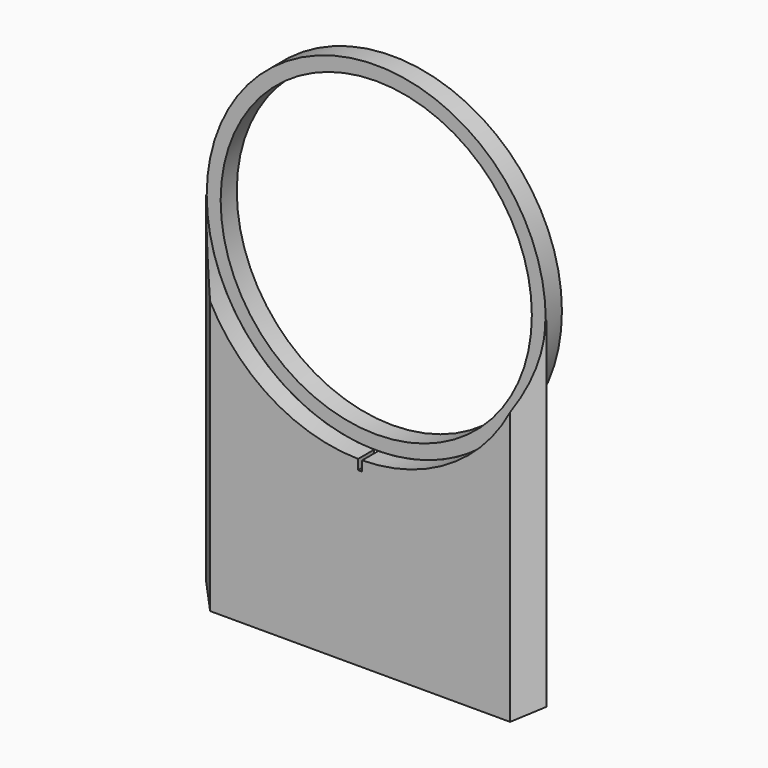
from build123d import *

# Parameters (mm, degrees)
F1_R         = 42.0358065459
F3_DEPTH     = 5
F2_R         = 38.5790977184
F4_DEPTH     = 5
F0_R         = 2
F5_DEPTH     = 25
F6_W         = 84.3785708158
F6_H         = 87.1892854079
F6_W_2       = 1
F6_H_2       = 5
F7_DEPTH     = 5
F8_DEPTH     = 5
F9_SIZE2     = 2.886741
F9_SIZE      = 4.99999
F10_T1_DEPTH = 112.9061152876


# Not quite as in the source:
# - a fillet or chamfer that OpenCascade refuses, or shapes differently, is made with other operations: its cross-section is extruded or revolved along the edge and cut away or added
# - a fillet or chamfer is up to 0.001 mm smaller than in the source, because OpenCascade refuses the exact size


with BuildPart() as f3:
    # F1 (on Front) → F3 (new body, symmetric)
    with BuildSketch(Plane.XZ):
        Circle(F1_R)
    extrude(amount=F3_DEPTH, both=True)

    # F2 (on Front) → F4 (cut)
    with BuildSketch(Plane.XZ):
        Circle(F2_R)
    extrude(amount=-F4_DEPTH, mode=Mode.SUBTRACT)

    # F0 (on Front) → F5 (cut)
    with BuildSketch(Plane.XZ):
        with BuildLine():
            ThreePointArc((26, 24), (24, 26), (22, 24))
            ThreePointArc((22, 24), (24, 22), (26, 24))
        make_face()
        with BuildLine():
            ThreePointArc((12.5, 24), (0, 27.0601182555), (-12.5, 24))
            Line((-12.5, 24), (12.5, 24))
        make_face()
        with BuildLine():
            Line((12.5, 24), (-12.5, 24))
            ThreePointArc((-12.5, 24), (-27.0601182555, 0), (-12.5, -24))
            Line((-12.5, -24), (12.5, -24))
            ThreePointArc((12.5, -24), (23.1354865757, -14.0356425184), (27.0601182555, 0))
            ThreePointArc((27.0601182555, 0), (23.1354865757, 14.0356425184), (12.5, 24))
        make_face()
        with Locations((-24, 24)):
            Circle(F0_R)
        with BuildLine():
            ThreePointArc((12.5, -24), (0, -27.0601182555), (-12.5, -24))
            Line((-12.5, -24), (-12.5, -28))
            Line((-12.5, -28), (12.5, -28))
            Line((12.5, -28), (12.5, -24))
        make_face()
        with BuildLine():
            Line((12.5, -24), (-12.5, -24))
            ThreePointArc((-12.5, -24), (0, -27.0601182555), (12.5, -24))
        make_face()
        with Locations((24, -24)):
            Circle(F0_R)
        with Locations((-24, -24)):
            Circle(F0_R)
    extrude(amount=F5_DEPTH, mode=Mode.SUBTRACT)


with BuildPart() as f7:
    # F6 (on Front) → F7 (new body)
    with BuildSketch(Plane.XZ):
        with Locations((0, -43.5946427039)):
            Rectangle(F6_W, F6_H)
        with Locations((0, -42)):
            Rectangle(F6_W_2, F6_H_2, mode=Mode.SUBTRACT)
    extrude(amount=F7_DEPTH)


with BuildPart() as f8_tool:
    # F1 (on Front) → F8 (new body)
    with BuildSketch(Plane.XZ):
        Circle(F1_R)
    extrude(amount=F8_DEPTH)


with BuildPart() as f3_1:
    add(f3.part)

    # F8: cut by f8_tool
    add(f8_tool.part, mode=Mode.SUBTRACT)


with BuildPart() as f7_1:
    add(f7.part)

    # F8: cut by f8_tool
    add(f8_tool.part, mode=Mode.SUBTRACT)

    # F9 (size 5 and 2.8867513459 in the source; OpenCascade refuses exactly that, so slightly less here)
    f9_edges = [f7_1.edges().sort_by_distance(p)[0] for p in [
        (0, 0, -87.189285),
    ]]
    f9_side = f7_1.faces().sort_by_distance((0, -2.5, -87.189285))[0]
    chamfer(f9_edges, length=F9_SIZE, length2=F9_SIZE2, reference=f9_side)

    # F10: chamfer of 5 on 2 edges, made by hand

    # F10_s2 → F10_t1 (cut)
    with BuildSketch(Plane.XY.offset(-100.0477003477)):
        Polygon((-42.1892854079, 0), (-37.1892854079, -5), (-42.1892854079, -5), align=None)
        Polygon((42.1892854079, 0), (37.1892854079, -5), (42.1892854079, -5), align=None)
    extrude(amount=F10_T1_DEPTH, mode=Mode.SUBTRACT)


solid = Compound([f3_1.part, f7_1.part])
